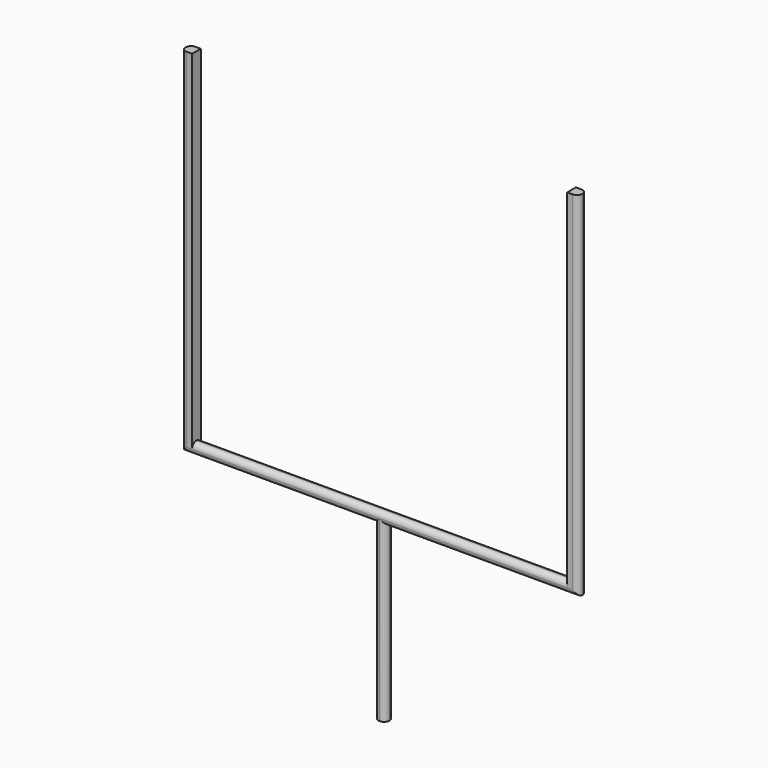
from build123d import *

# Parameters (mm, degrees)
F1_DEPTH = 9.525
F2_R     = 4.76249


# Not quite as in the source:
# - a fillet or chamfer is up to 0.001 mm smaller than in the source, because OpenCascade refuses the exact size


with BuildPart() as f1:
    # F0 (on Front) → F1 (new body)
    with BuildSketch(Plane.XZ):
        Polygon((-9.3524411189, 93.575365177), (-9.3524411189, -58.8385015355), (-4.5891202249, -58.8385015355), (0.174200669, -58.8385015355), (0.174200669, 93.575365177), (170.0456099196, 93.575365177), (170.0456099196, 404.7306356684), (160.5287608864, 404.7306356684), (160.5287608864, 103.1056356684), (-4.5891202249, 103.1056356684), (-169.7070013363, 103.1056356684), (-169.7070013363, 404.7306356684), (-179.2238503695, 404.7306356684), (-179.2238503695, 93.575365177), align=None)
    extrude(amount=F1_DEPTH)

    # F2 (radius 4.7625 in the source; OpenCascade refuses exactly that, so slightly less here)
    f2_edges = [f1.edges().sort_by_distance(p)[0] for p in [
        (170.04561, -9.525, 249.153),
        (170.04561, 0, 249.153),
        (-4.58912, 0, 103.105636),
        (-4.58912, -9.525, 103.105636),
        (-94.288146, -9.525, 93.575365),
        (-94.288146, 0, 93.575365),
        (85.109905, -9.525, 93.575365),
        (85.109905, 0, 93.575365),
        (0.174201, -9.525, 17.368432),
        (-9.352441, -9.525, 17.368432),
        (-9.352441, 0, 17.368432),
        (0.174201, 0, 17.368432),
        (-179.22385, 0, 249.153),
        (-179.22385, -9.525, 249.153),
    ]]
    fillet(f2_edges, radius=F2_R)


solid = f1.part
